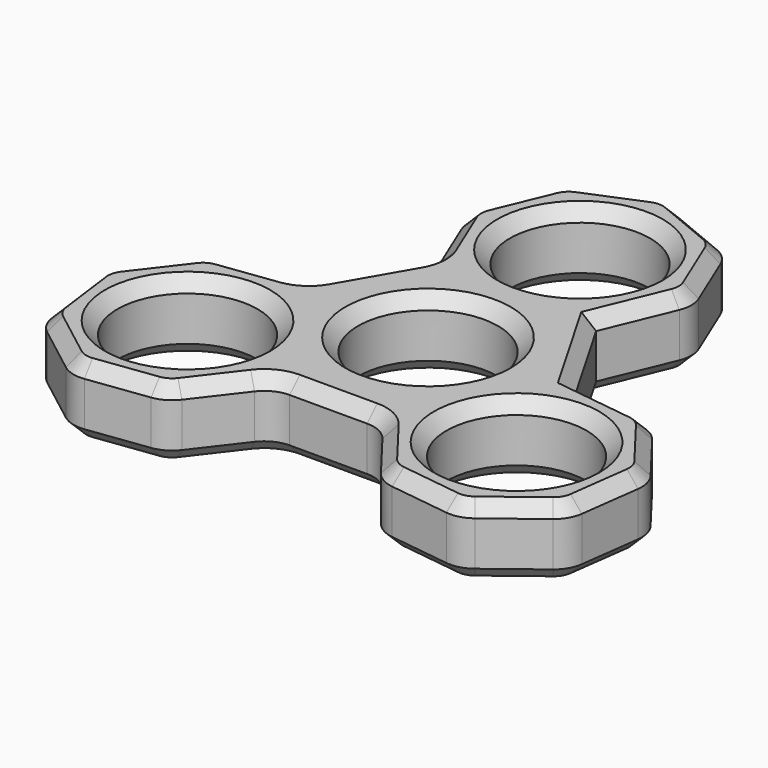
from build123d import *

# Parameters (mm, degrees)
F0_R     = 11.0625
F1_DEPTH = 11
F2_R     = 5
F3_SIZE  = 2
F4_SIZE  = 2


# Not quite as in the source:
# - a feature names something its author has since deleted; it is built from what else it names


with BuildPart() as f1:
    # F0 (on Top) → F1 (new body)
    with BuildSketch(Plane.XY):
        Polygon((12.7279220614, 42.7279220614), (0, 48), (-12.7279220614, 42.7279220614), (-18, 30), (-12.7279220614, 17.2720779386), (-21.3220193017, 2.3866648732), (-34.9807621135, 0.5884572681), (-43.3674269867, -10.3412571882), (-41.5692193817, -24), (-30.6395049254, -32.3866648732), (-16.9807621135, -30.5884572681), (-8.5940972403, -19.6587428118), (8.5940972403, -19.6587428118), (16.9807621135, -30.5884572681), (30.6395049254, -32.3866648732), (41.5692193817, -24), (43.3674269867, -10.3412571882), (34.9807621135, 0.5884572681), (21.3220193017, 2.3866648732), (12.7279220614, 17.2720779386), (18, 30), align=None)
        with Locations((-25.9807621135, -15)):
            Circle(F0_R, mode=Mode.SUBTRACT)
        Circle(F0_R, mode=Mode.SUBTRACT)
        with Locations((25.9807621135, -15)):
            Circle(F0_R, mode=Mode.SUBTRACT)
        with Locations((0, 30)):
            Circle(F0_R, mode=Mode.SUBTRACT)
    extrude(amount=F1_DEPTH)

    # F2
    f2_edges = [f1.edges().sort_by_distance(p)[0] for p in [
        (-16.980762, -30.588457, 5.5),
        (-30.639505, -32.386665, 5.5),
        (-41.569219, -24, 5.5),
        (-43.367427, -10.341257, 5.5),
        (-34.980762, 0.588457, 5.5),
        (-18, 30, 5.5),
        (-12.727922, 42.727922, 5.5),
        (0, 48, 5.5),
        (12.727922, 42.727922, 5.5),
        (34.980762, 0.588457, 5.5),
        (43.367427, -10.341257, 5.5),
        (41.569219, -24, 5.5),
        (30.639505, -32.386665, 5.5),
        (16.980762, -30.588457, 5.5),
        (8.594097, -19.658743, 5.5),
        (-8.594097, -19.658743, 5.5),
        (18, 30, 5.5),
        (-12.727922, 17.272078, 5.5),
        (-21.322019, 2.386665, 5.5),
    ]]
    fillet(f2_edges, radius=F2_R)

    # F3
    f3_edges = [f1.edges().sort_by_distance(p)[0] for p in [
        (27.124716, 1.622725, 11),
        (34.774782, 0.231689, 11),
        (17.024971, 9.829371, 11),
        (39.174095, -4.8764, 11),
        (14.967679, 22.67933, 11),
        (42.969503, -10.447881, 11),
        (17.588039, 30, 11),
        (42.468323, -17.170629, 11),
        (15.363961, 36.363961, 11),
        (41.212451, -23.794019, 11),
        (12.436622, 42.436622, 11),
        (36.104362, -28.193332, 11),
        (6.363961, 45.363961, 11),
        (30.532882, -31.988741, 11),
        (0, 47.588039, 11),
        (23.810134, -31.487561, 11),
        (-6.363961, 45.363961, 11),
        (17.186743, -30.231689, 11),
        (-12.436622, 42.436622, 11),
        (12.907556, -25.280152, 11),
        (-15.363961, 36.363961, 11),
        (8.339814, -20.174379, 11),
        (-17.588039, 30, 11),
        (0, -19.658743, 11),
        (-15.439476, 23.818348, 11),
        (-8.339814, -20.174379, 11),
        (-13.301618, 17.30968, 11),
        (-12.907556, -25.280152, 11),
        (-17.024971, 9.829371, 11),
        (-17.186743, -30.231689, 11),
        (-21.641432, 2.864699, 11),
        (-23.810134, -31.487561, 11),
        (-28.347032, 1.461804, 11),
        (-30.532882, -31.988741, 11),
        (-34.774782, 0.231689, 11),
        (-36.104362, -28.193332, 11),
        (-39.174095, -4.8764, 11),
        (-41.212451, -23.794019, 11),
        (-42.969503, -10.447881, 11),
        (-42.468323, -17.170629, 11),
        (-37.043262, -15, 11),
        (-11.0625, 0, 11),
        (14.918262, -15, 11),
        (-11.0625, 30, 11),
    ]]
    chamfer(f3_edges, length=F3_SIZE)

    # F4
    f4_edges = [f1.edges().sort_by_distance(p)[0] for p in [
        (27.124716, 1.622725, 0),
        (34.774782, 0.231689, 0),
        (17.024971, 9.829371, 0),
        (39.174095, -4.8764, 0),
        (14.967679, 22.67933, 0),
        (42.969503, -10.447881, 0),
        (17.588039, 30, 0),
        (42.468323, -17.170629, 0),
        (15.363961, 36.363961, 0),
        (41.212451, -23.794019, 0),
        (12.436622, 42.436622, 0),
        (36.104362, -28.193332, 0),
        (6.363961, 45.363961, 0),
        (30.532882, -31.988741, 0),
        (0, 47.588039, 0),
        (23.810134, -31.487561, 0),
        (-6.363961, 45.363961, 0),
        (17.186743, -30.231689, 0),
        (-12.436622, 42.436622, 0),
        (12.907556, -25.280152, 0),
        (-15.363961, 36.363961, 0),
        (8.339814, -20.174379, 0),
        (-17.588039, 30, 0),
        (0, -19.658743, 0),
        (-15.439476, 23.818348, 0),
        (-8.339814, -20.174379, 0),
        (-13.301618, 17.30968, 0),
        (-12.907556, -25.280152, 0),
        (-17.024971, 9.829371, 0),
        (-17.186743, -30.231689, 0),
        (-21.641432, 2.864699, 0),
        (-23.810134, -31.487561, 0),
        (-28.347032, 1.461804, 0),
        (-30.532882, -31.988741, 0),
        (-34.774782, 0.231689, 0),
        (-36.104362, -28.193332, 0),
        (-39.174095, -4.8764, 0),
        (-41.212451, -23.794019, 0),
        (-42.969503, -10.447881, 0),
        (-42.468323, -17.170629, 0),
        (-37.043262, -15, 0),
        (-11.0625, 0, 0),
        (14.918262, -15, 0),
        (-11.0625, 30, 0),
    ]]
    chamfer(f4_edges, length=F4_SIZE)


solid = f1.part
